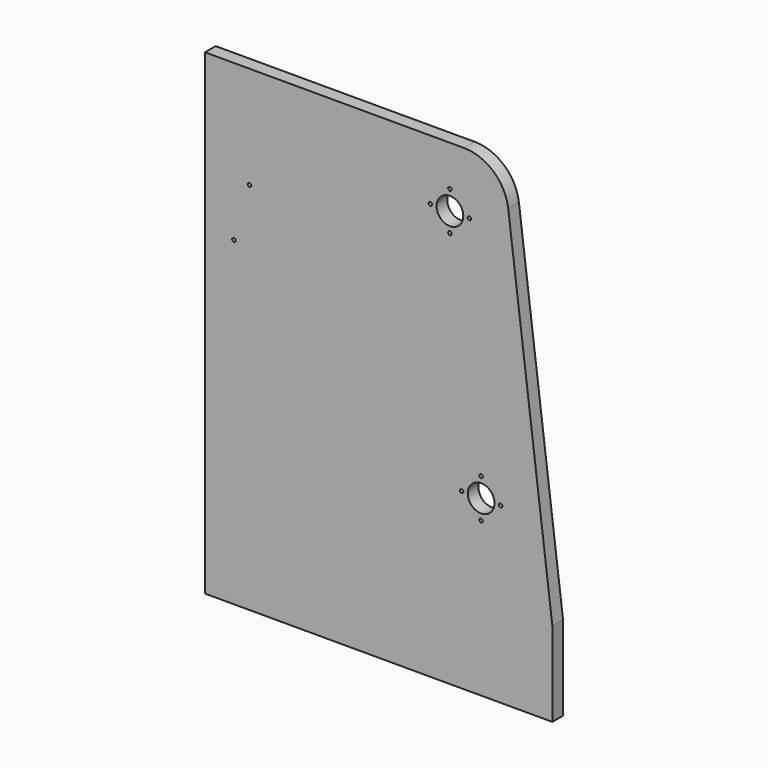
from build123d import *

# Parameters (mm, degrees)
F0_R     = 38.1
F1_DEPTH = 38.1
F3_D     = 10.0838


# Not quite as in the source:
# - a feature names something its author has since deleted; it is built from what else it names


with BuildPart() as f1:
    # F0 (on Front) → F1 (new body)
    with BuildSketch(Plane.XZ):
        with BuildLine():
            Line((0, 1358.9), (0, 0))
            Line((0, 0), (990.6, 0))
            Line((990.6, 0), (990.6, 241.3))
            Line((990.6, 241.3), (864.8059485884, 1247.6524112928))
            ThreePointArc((864.8059485884, 1247.6524112928), (822.8355837767, 1327.1091283286), (738.7866582458, 1358.9))
            Line((738.7866582458, 1358.9), (0, 1358.9))
        make_face()
        with Locations((787.4, 495.3)):
            Circle(F0_R, mode=Mode.SUBTRACT)
        with Locations((698.5, 1187.45)):
            Circle(F0_R, mode=Mode.SUBTRACT)
    extrude(amount=F1_DEPTH)

    # F3 (through all)
    with Locations(Plane.XZ.offset(38.1)):
        with Locations((82.55, 914.4), (127, 1066.8), (698.5, 1243.0125), (754.0625, 1187.45), (698.5, 1131.8875), (642.9375, 1187.45), (842.9625, 495.3), (787.4, 550.8625), (731.8375, 495.3), (787.4, 439.7375)):
            Hole(F3_D / 2)


solid = f1.part
